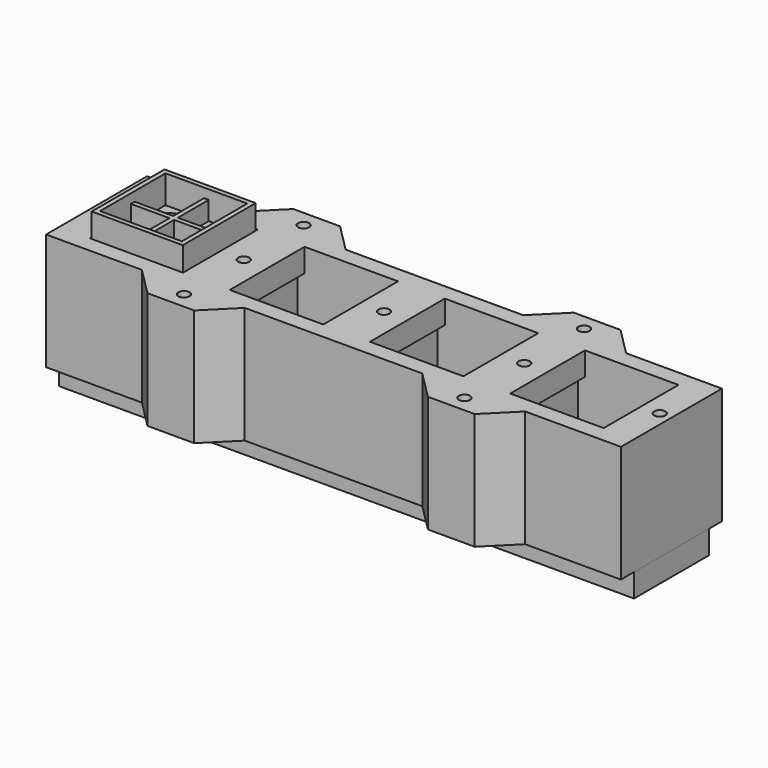
from build123d import *

# Parameters (mm, degrees)
F0_W      = 19.5
F0_H      = 19.5
F1_DEPTH  = 13
F2_W      = 19.5
F2_H      = 19.5
F2_W_2    = 17.5
F2_H_2    = 17.5
F3_DEPTH  = 6
F5_DEPTH  = 4
F6_R      = 3.1
F7_DEPTH  = 19
F8_W      = 1.5
F8_H      = 19.5
F9_DEPTH  = 9
F10_R     = 2.55
F11_DEPTH = 3
F13_W     = 10
F13_H     = 6
F13_W_2   = 20
F13_H_2   = 20
F14_DEPTH = 25
F15_W     = 23
F15_H     = 20
F16_DEPTH = 20
F17_R     = 1.2
F18_DEPTH = 30
F19_R     = 1.2
F20_DEPTH = 30.001
F21_W     = 123
F21_H     = 20
F21_R     = 2.75
F21_R_2   = 1.5
F21_R_3   = 4
F22_DEPTH = 5
F23_SIZE  = 5.99999
F25_W     = 3
F25_H     = 8
F25_H_2   = 3
F25_W_2   = 9.5
F26_DEPTH = 10.5


# Not quite as in the source:
# - a fillet or chamfer is up to 0.001 mm smaller than in the source, because OpenCascade refuses the exact size


with BuildPart() as f1:
    # F0 (on Top) → F1 (new body)
    with BuildSketch(Plane.XY):
        Rectangle(F0_W, F0_H)
    extrude(amount=F1_DEPTH)

    # F2 (on face) → F3 (join)
    with BuildSketch(Plane.XY.offset(13)):
        Rectangle(F2_W, F2_H)
        Rectangle(F2_W_2, F2_H_2, mode=Mode.SUBTRACT)
    extrude(amount=F3_DEPTH)

    # F4 (on face) → F5 (join)
    with BuildSketch(Plane.XY.offset(13)):
        Polygon((0.5, 8.75), (-0.5, 8.75), (-0.5, 0.5), (-8.75, 0.5), (-8.75, -0.5), (-0.5, -0.5), (-0.5, -8.75), (0.5, -8.75), (0.5, -0.5), (8.75, -0.5), (8.75, 0.5), (0.5, 0.5), align=None)
    extrude(amount=F5_DEPTH)

    # F6 (on face) → F7 (cut)
    with BuildSketch(Plane.XY.offset(13)):
        with Locations((-4.5, 4.5)):
            Circle(F6_R)
        with Locations((-4.5, -4.5)):
            Circle(F6_R)
        with Locations((4.5, 4.5)):
            Circle(F6_R)
        with Locations((4.5, -4.5)):
            Circle(F6_R)
    extrude(amount=-F7_DEPTH, mode=Mode.SUBTRACT)

    # F8 (on face) → F9 (join)
    with BuildSketch(Plane(origin=(0, 0, 0), x_dir=(1, 0, 0), z_dir=(0, 0, -1))):
        with Locations((-10.5, 0)):
            Rectangle(F8_W, F8_H)
        with Locations((10.5, 0)):
            Rectangle(F8_W, F8_H)
    extrude(amount=-F9_DEPTH)

    # F10 (on face) → F11 (cut)
    with BuildSketch(Plane(origin=(0, 0, 0), x_dir=(1, 0, 0), z_dir=(0, 0, -1))):
        Circle(F10_R)
    extrude(amount=-F11_DEPTH, mode=Mode.SUBTRACT)


with BuildPart() as f14:
    # F13 (on offset) → F14 (new body)
    with BuildSketch(Plane.XY.offset(14)):
        with Locations((15, 16.5)):
            Rectangle(F13_W, F13_H)
        Polygon((20, 13.5), (10, 13.5), (-16.5, 13.5), (-16.5, -13.5), (10, -13.5), (20, -13.5), (70, -13.5), (80, -13.5), (106.5, -13.5), (106.5, 13.5), (80, 13.5), (70, 13.5), align=None)
        Rectangle(F13_W_2, F13_H_2, mode=Mode.SUBTRACT)
        with Locations((30, 0)):
            Rectangle(F13_W_2, F13_H_2, mode=Mode.SUBTRACT)
        with Locations((60, 0)):
            Rectangle(F13_W_2, F13_H_2, mode=Mode.SUBTRACT)
        with Locations((90, 0)):
            Rectangle(F13_W_2, F13_H_2, mode=Mode.SUBTRACT)
        with Locations((75, 16.5)):
            Rectangle(F13_W, F13_H)
        with Locations((15, -16.5)):
            Rectangle(F13_W, F13_H)
        with Locations((75, -16.5)):
            Rectangle(F13_W, F13_H)
    extrude(amount=-F14_DEPTH)

    # F15 (on face) → F16 (cut)
    with BuildSketch(Plane(origin=(0, 0, -11), x_dir=(1, 0, 0), z_dir=(0, 0, -1))):
        Rectangle(F15_W, F15_H)
        with Locations((30, 0)):
            Rectangle(F15_W, F15_H)
        with Locations((60, 0)):
            Rectangle(F15_W, F15_H)
        with Locations((90, 0)):
            Rectangle(F15_W, F15_H)
    extrude(amount=-F16_DEPTH, mode=Mode.SUBTRACT)

    # F17 (on face) → F18 (cut)
    with BuildSketch(Plane.XY.offset(14)):
        with Locations((15, 16)):
            Circle(F17_R)
        with Locations((15, -16)):
            Circle(F17_R)
        with Locations((75, 16)):
            Circle(F17_R)
        with Locations((75, -16)):
            Circle(F17_R)
    extrude(amount=-F18_DEPTH, mode=Mode.SUBTRACT)

    # F19 (on face) → F20 (cut, through all)
    with BuildSketch(Plane(origin=(0, 0, -11), x_dir=(1, 0, 0), z_dir=(0, 0, -1))):
        with Locations((-14, 0)):
            Circle(F19_R)
        with Locations((15, 0)):
            Circle(F19_R)
        with Locations((45, 0)):
            Circle(F19_R)
        with Locations((75, 0)):
            Circle(F19_R)
        with Locations((104, 0)):
            Circle(F19_R)
    extrude(amount=-F20_DEPTH, mode=Mode.SUBTRACT)

    # F23 (size 6 in the source; OpenCascade refuses exactly that, so slightly less here)
    f23_edges = [f14.edges().sort_by_distance(p)[0] for p in [
        (10, -13.5, 1.5),
        (20, -13.5, 1.5),
        (70, -13.5, 1.5),
        (80, -13.5, 1.5),
        (10, 13.5, 1.5),
        (20, 13.5, 1.5),
        (70, 13.5, 1.5),
        (80, 13.5, 1.5),
    ]]
    chamfer(f23_edges, length=F23_SIZE)


with BuildPart() as f22:
    # F21 (on face) → F22 (new body)
    with BuildSketch(Plane(origin=(0, 0, -11), x_dir=(1, 0, 0), z_dir=(0, 0, -1))):
        with Locations((45, 0)):
            Rectangle(F21_W, F21_H)
        with Locations((-5.5, -5.5)):
            Circle(F21_R, mode=Mode.SUBTRACT)
        with Locations((5.5, -5.5)):
            Circle(F21_R, mode=Mode.SUBTRACT)
        with Locations((24.5, -5.5)):
            Circle(F21_R, mode=Mode.SUBTRACT)
        with Locations((35.5, -5.5)):
            Circle(F21_R, mode=Mode.SUBTRACT)
        with Locations((54.5, -5.5)):
            Circle(F21_R, mode=Mode.SUBTRACT)
        with Locations((65.5, -5.5)):
            Circle(F21_R, mode=Mode.SUBTRACT)
        with Locations((84.5, -5.5)):
            Circle(F21_R, mode=Mode.SUBTRACT)
        with Locations((95.5, -5.5)):
            Circle(F21_R, mode=Mode.SUBTRACT)
        with Locations((-14, 0)):
            Circle(F21_R_2, mode=Mode.SUBTRACT)
        Circle(F21_R_3, mode=Mode.SUBTRACT)
        with Locations((15, 0)):
            Circle(F21_R_2, mode=Mode.SUBTRACT)
        with Locations((30, 0)):
            Circle(F21_R_3, mode=Mode.SUBTRACT)
        with Locations((-5.5, 5.5)):
            Circle(F21_R, mode=Mode.SUBTRACT)
        with Locations((5.5, 5.5)):
            Circle(F21_R, mode=Mode.SUBTRACT)
        with Locations((24.5, 5.5)):
            Circle(F21_R, mode=Mode.SUBTRACT)
        with Locations((35.5, 5.5)):
            Circle(F21_R, mode=Mode.SUBTRACT)
        with Locations((45, 0)):
            Circle(F21_R_2, mode=Mode.SUBTRACT)
        with Locations((60, 0)):
            Circle(F21_R_3, mode=Mode.SUBTRACT)
        with Locations((75, 0)):
            Circle(F21_R_2, mode=Mode.SUBTRACT)
        with Locations((90, 0)):
            Circle(F21_R_3, mode=Mode.SUBTRACT)
        with Locations((104, 0)):
            Circle(F21_R_2, mode=Mode.SUBTRACT)
        with Locations((54.5, 5.5)):
            Circle(F21_R, mode=Mode.SUBTRACT)
        with Locations((65.5, 5.5)):
            Circle(F21_R, mode=Mode.SUBTRACT)
        with Locations((84.5, 5.5)):
            Circle(F21_R, mode=Mode.SUBTRACT)
        with Locations((95.5, 5.5)):
            Circle(F21_R, mode=Mode.SUBTRACT)
    extrude(amount=F22_DEPTH)


with BuildPart() as f26:
    # F25 (on offset) → F26 (new body)
    with BuildSketch(Plane(origin=(0, 0, -11), x_dir=(1, 0, 0), z_dir=(0, 0, -1))):
        with Locations((0, -5.5)):
            Rectangle(F25_W, F25_H)
        Rectangle(F25_W, F25_H_2)
        with Locations((6.25, 0)):
            Rectangle(F25_W_2, F25_H_2)
        with Locations((-6.25, 0)):
            Rectangle(F25_W_2, F25_H_2)
        with Locations((0, 5.5)):
            Rectangle(F25_W, F25_H)
    extrude(amount=-F26_DEPTH)


solid = Compound([f1.part, f14.part, f22.part, f26.part])
